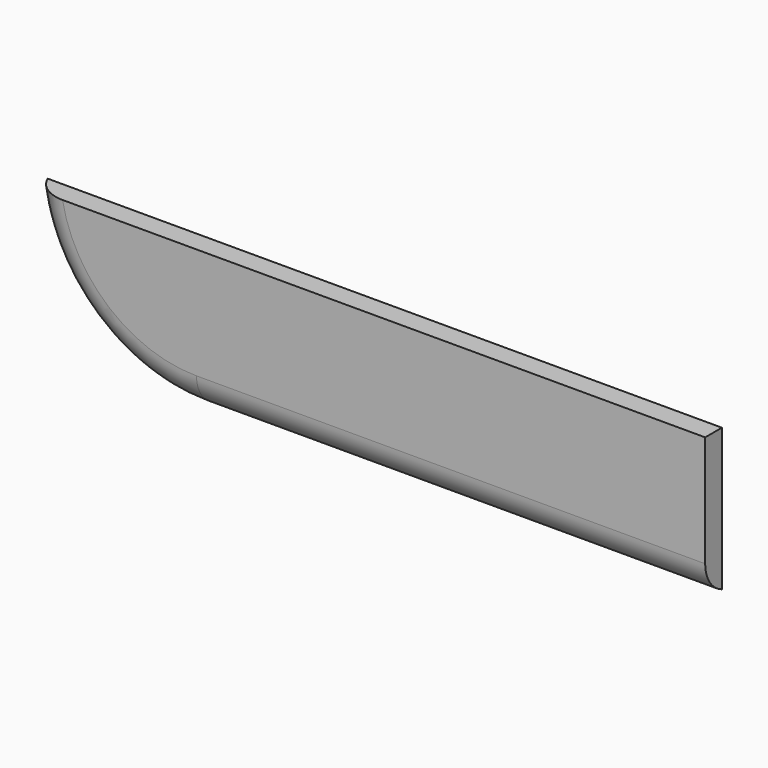
from build123d import *

# Parameters (mm, degrees)
F1_DEPTH    = 3.175
F2_T1_DEPTH = 88.9594546746
F2_T4_ANGLE = 107.955272034


# Not quite as in the source:
# - a fillet or chamfer that OpenCascade refuses, or shapes differently, is made with other operations: its cross-section is extruded or revolved along the edge and cut away or added


with BuildPart() as f1:
    # F0 (on Front) → F1 (new body)
    with BuildSketch(Plane.XZ):
        with BuildLine():
            Line((-25.8931197882, -10.7985436916), (51.2931197882, -10.7985436916))
            Line((51.2931197882, -10.7985436916), (51.2931197882, 10.7985436916))
            Line((51.2931197882, 10.7985436916), (-51.0068183535, 10.7985436916))
            ThreePointArc((-51.0068183535, 10.7985436916), (-42.4546115618, -4.6567105367), (-25.8931197882, -10.7985436916))
        make_face()
    extrude(amount=F1_DEPTH)

    # F2: fillet of radius 5.08 on 1 edges, made by hand

    # F2_s2 → F2_t1 (cut)
    with BuildSketch(Plane.YZ.offset(-25.8931197882)):
        with BuildLine():
            ThreePointArc((0, -10.7985436916), (-2.3071134838, -8.9290639838), (-3.175, -6.0892576523))
            Line((-3.175, -6.0892576523), (-3.175, -10.7985436916))
            Line((-3.175, -10.7985436916), (0, -10.7985436916))
        make_face()
    extrude(amount=F2_T1_DEPTH, mode=Mode.SUBTRACT)

    # F2_s3 → F2_t4 (revolve, cut)
    with BuildSketch(Plane(origin=(1.8213289156, 0, 5.6203993841), x_dir=(0, 1, 0), z_dir=(0.3082744578, 0, 0.9512974607))):
        with BuildLine():
            ThreePointArc((0, 54.5333151295), (-2.3071134838, 52.6638354216), (-3.175, 49.8240290902))
            Line((-3.175, 49.8240290902), (-3.175, 54.5333151295))
            Line((-3.175, 54.5333151295), (0, 54.5333151295))
        make_face()
    revolve(axis=Axis((-25.8931197882, -3.175, 14.6014563084), (0, -1, 0)), revolution_arc=F2_T4_ANGLE, mode=Mode.SUBTRACT)


solid = f1.part
